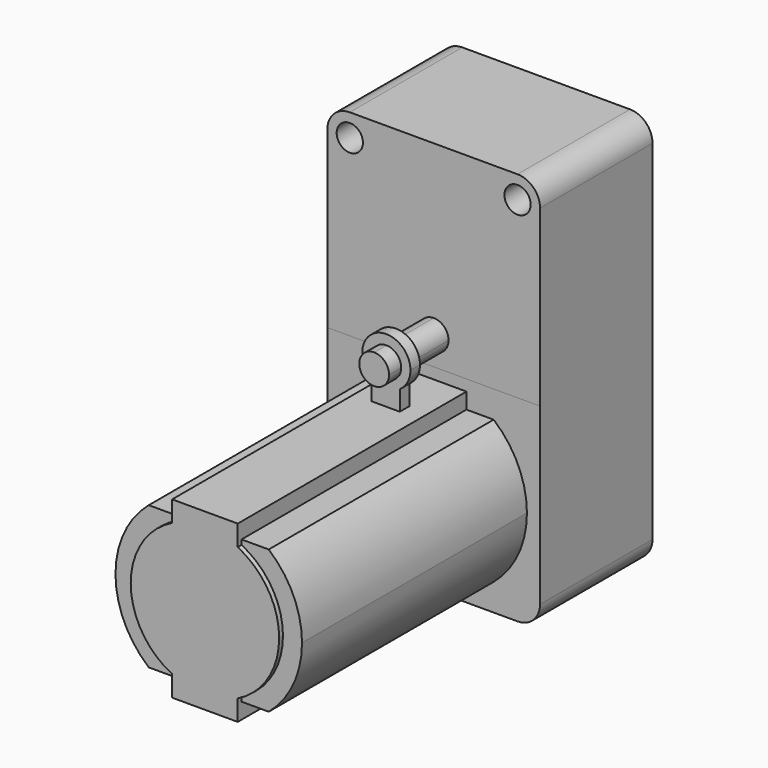
from build123d import *

# Parameters (mm, degrees)
F0_W      = 22.7
F0_H      = 15
F1_DEPTH  = 42
F0_H_2    = 30
F2_DEPTH  = 21
F4_DEPTH  = 7.9375
F5_R      = 2.4
F8_DEPTH  = 29.99994
F11_DEPTH = 1.27
F12_R     = 2.3876
F13_DEPTH = 8.001
F14_DEPTH = 0.762
F6_R      = 1.4
F15_DEPTH = 25.4
F16_DEPTH = 0.508


# Not quite as in the source:
# - a length typed as a fraction of an inch, garbled in the dataset ("3 / 203.2 mm" for 3/8 in), is restored


with BuildPart() as f1:
    # F0 (on Top) → F1 (new body)
    with BuildSketch(Plane.XY):
        with Locations((0, 15)):
            Rectangle(F0_W, F0_H)
    extrude(amount=F1_DEPTH)

    # F0 (on Top) → F2 (join)
    with BuildSketch(Plane.XY):
        with Locations((0, 15)):
            Rectangle(F0_W, F0_H)
        with Locations((0, -7.5)):
            Rectangle(F0_W, F0_H_2)
    extrude(amount=F2_DEPTH)

    # F3 (on face) → F4 (join)
    with BuildSketch(Plane.XZ.offset(-7.5)):
        with BuildLine():
            Line((0, 25.5875), (0, 22.4125))
            ThreePointArc((0, 22.4125), (1.1225320151, 22.8774679849), (1.5875, 24))
            ThreePointArc((1.5875, 24), (1.1225320151, 25.1225320151), (0, 25.5875))
        make_face()
        with BuildLine():
            ThreePointArc((0, 25.5875), (-1.5875, 24), (0, 22.4125))
            Line((0, 22.4125), (0, 25.5875))
        make_face()
    extrude(amount=F4_DEPTH)

    # F5
    f5_edges = [f1.edges().sort_by_distance(p)[0] for p in [
        (-11.35, 15, 42),
        (11.35, 15, 42),
    ]]
    fillet(f5_edges, radius=F5_R)

    # F7 (on face) → F8 (cut)
    with BuildSketch(Plane.XZ.offset(22.5)):
        with BuildLine():
            Line((11.35, 21), (0, 21))
            Line((0, 21), (0, 20.45045))
            ThreePointArc((0, 20.45045), (1.7780416897, 20.2903024954), (3.49885, 19.8150149694))
            ThreePointArc((3.49885, 19.8150149694), (5.0209631758, 19.0907731893), (6.3989886078, 18.12))
            ThreePointArc((6.3989886078, 18.12), (9.0189875095, 14.7034889681), (9.95045, 10.5))
            Line((9.95045, 10.5), (11.35, 10.5))
            Line((11.35, 10.5), (11.35, 21))
        make_face()
        with BuildLine():
            Line((0, 20.45045), (0, 21))
            Line((0, 21), (-11.35, 21))
            Line((-11.35, 21), (-11.35, 10.5))
            Line((-11.35, 10.5), (-9.95045, 10.5))
            ThreePointArc((-9.95045, 10.5), (-9.0189875095, 14.7034889681), (-6.3989886078, 18.12))
            ThreePointArc((-6.3989886078, 18.12), (-5.0209631758, 19.0907731893), (-3.49885, 19.8150149694))
            ThreePointArc((-3.49885, 19.8150149694), (-1.7780416897, 20.2903024954), (0, 20.45045))
        make_face()
        with BuildLine():
            Line((-3.49885, 18.12), (-3.49885, 19.8150149694))
            ThreePointArc((-3.49885, 19.8150149694), (-5.0209631758, 19.0907731893), (-6.3989886078, 18.12))
            Line((-6.3989886078, 18.12), (-3.49885, 18.12))
        make_face()
        with BuildLine():
            ThreePointArc((6.3989886078, 18.12), (5.0209631758, 19.0907731893), (3.49885, 19.8150149694))
            Line((3.49885, 19.8150149694), (3.49885, 18.12))
            Line((3.49885, 18.12), (6.3989886078, 18.12))
        make_face()
        with BuildLine():
            Line((-9.95045, 10.5), (-11.35, 10.5))
            Line((-11.35, 10.5), (-11.35, 0))
            Line((-11.35, 0), (0, 0))
            Line((0, 0), (0, 0.54955))
            ThreePointArc((0, 0.54955), (-1.7780416897, 0.7096975046), (-3.49885, 1.1849850306))
            ThreePointArc((-3.49885, 1.1849850306), (-5.0209631758, 1.9092268107), (-6.3989886078, 2.88))
            ThreePointArc((-6.3989886078, 2.88), (-9.0189875095, 6.2965110319), (-9.95045, 10.5))
        make_face()
        with BuildLine():
            Line((11.35, 0), (11.35, 10.5))
            Line((11.35, 10.5), (9.95045, 10.5))
            ThreePointArc((9.95045, 10.5), (9.0189875095, 6.2965110319), (6.3989886078, 2.88))
            ThreePointArc((6.3989886078, 2.88), (5.0209631758, 1.9092268107), (3.49885, 1.1849850306))
            ThreePointArc((3.49885, 1.1849850306), (1.7780416897, 0.7096975046), (0, 0.54955))
            Line((0, 0.54955), (0, 0))
            Line((0, 0), (11.35, 0))
        make_face()
        with BuildLine():
            ThreePointArc((3.49885, 1.1849850306), (5.0209631758, 1.9092268107), (6.3989886078, 2.88))
            Line((6.3989886078, 2.88), (3.49885, 2.88))
            Line((3.49885, 2.88), (3.49885, 1.1849850306))
        make_face()
        with BuildLine():
            Line((-3.49885, 2.88), (-6.3989886078, 2.88))
            ThreePointArc((-6.3989886078, 2.88), (-5.0209631758, 1.9092268107), (-3.49885, 1.1849850306))
            Line((-3.49885, 1.1849850306), (-3.49885, 2.88))
        make_face()
        with BuildLine():
            ThreePointArc((3.49885, 19.8150149694), (1.7780416897, 20.2903024954), (0, 20.45045))
            Line((0, 20.45045), (0, 19.8150149694))
            Line((0, 19.8150149694), (3.49885, 19.8150149694))
        make_face()
        with BuildLine():
            Line((0, 19.8150149694), (0, 20.45045))
            ThreePointArc((0, 20.45045), (-1.7780416897, 20.2903024954), (-3.49885, 19.8150149694))
            Line((-3.49885, 19.8150149694), (0, 19.8150149694))
        make_face()
        with BuildLine():
            ThreePointArc((0, 0.54955), (1.7780416897, 0.7096975046), (3.49885, 1.1849850306))
            Line((3.49885, 1.1849850306), (0, 1.1849850306))
            Line((0, 1.1849850306), (0, 0.54955))
        make_face()
        with BuildLine():
            ThreePointArc((-3.49885, 1.1849850306), (-1.7780416897, 0.7096975046), (0, 0.54955))
            Line((0, 0.54955), (0, 1.1849850306))
            Line((0, 1.1849850306), (-3.49885, 1.1849850306))
        make_face()
    extrude(amount=-F8_DEPTH, mode=Mode.SUBTRACT)

    # F10 (on offset) → F11 (join)
    with BuildSketch(Plane.XZ.offset(-2.4581)):
        with BuildLine():
            ThreePointArc((1.4326738892, 21.9412771473), (2.2677347419, 22.8658808954), (2.5697519674, 24.0746010095))
            ThreePointArc((2.5697519674, 24.0746010095), (-1.1220643914, 26.3864393852), (-1.5898686834, 22.0557045923))
            Line((-1.5898686834, 22.0557045923), (-1.5898686834, 23.8072182983))
            Line((-1.5898686834, 23.8072182983), (1.4326738892, 23.8072182983))
            Line((1.4326738892, 23.8072182983), (1.4326738892, 21.9412771473))
        make_face()
        with BuildLine():
            Line((-1.5898686834, 23.8072182983), (-1.5898686834, 22.0557045923))
            ThreePointArc((-1.5898686834, 22.0557045923), (-0.0972160525, 21.5066885864), (1.4326738892, 21.9412771473))
            Line((1.4326738892, 21.9412771473), (1.4326738892, 23.8072182983))
            Line((1.4326738892, 23.8072182983), (-1.5898686834, 23.8072182983))
        make_face()
        with BuildLine():
            ThreePointArc((1.4326738892, 21.9412771473), (-0.0972160525, 21.5066885864), (-1.5898686834, 22.0557045923))
            Line((-1.5898686834, 22.0557045923), (-1.5898686834, 19.2958321422))
            Line((-1.5898686834, 19.2958321422), (1.4326738892, 19.2958321422))
            Line((1.4326738892, 19.2958321422), (1.4326738892, 21.9412771473))
        make_face()
    extrude(amount=F11_DEPTH)

    # F12
    f12_edges = [f1.edges().sort_by_distance(p)[0] for p in [
        (11.35, 14.99997, 0),
        (-11.35, 14.99997, 0),
    ]]
    fillet(f12_edges, radius=F12_R)

    # F6 (on face) → F13 (join)
    with BuildSketch(Plane(origin=(0, 22.5, 0), x_dir=(-1, 0, 0), z_dir=(0, 1, 0))):
        with BuildLine():
            ThreePointArc((1.86055, 32.8250564677), (0.9983973943, 33.3623627072), (0, 33.55))
            Line((0, 33.55), (0, 28.05))
            ThreePointArc((0, 28.05), (0.9983973943, 28.2376372928), (1.86055, 28.7749435323))
            Line((1.86055, 28.7749435323), (1.86055, 32.8250564677))
        make_face()
        with BuildLine():
            Line((0, 28.05), (0, 33.55))
            ThreePointArc((0, 33.55), (-0.9983973943, 33.3623627072), (-1.86055, 32.8250564677))
            Line((-1.86055, 32.8250564677), (-1.86055, 28.7749435323))
            ThreePointArc((-1.86055, 28.7749435323), (-0.9983973943, 28.2376372928), (0, 28.05))
        make_face()
    extrude(amount=F13_DEPTH)

    # F6 (on face) → F14 (join)
    with BuildSketch(Plane(origin=(0, 22.5, 0), x_dir=(-1, 0, 0), z_dir=(0, 1, 0))):
        with BuildLine():
            ThreePointArc((3.3400836906, 30.8), (2.3617958273, 33.1617958273), (0, 34.1400836906))
            Line((0, 34.1400836906), (0, 33.55))
            ThreePointArc((0, 33.55), (0.9983973943, 33.3623627072), (1.86055, 32.8250564677))
            ThreePointArc((1.86055, 32.8250564677), (2.5178376139, 31.9058904783), (2.75, 30.8))
            ThreePointArc((2.75, 30.8), (2.5178376139, 29.6941095217), (1.86055, 28.7749435323))
            ThreePointArc((1.86055, 28.7749435323), (0.9983973943, 28.2376372928), (0, 28.05))
            Line((0, 28.05), (0, 27.4599163094))
            ThreePointArc((0, 27.4599163094), (2.3617958273, 28.4382041727), (3.3400836906, 30.8))
        make_face()
        with BuildLine():
            Line((0, 33.55), (0, 34.1400836906))
            ThreePointArc((0, 34.1400836906), (-3.3400836906, 30.8), (0, 27.4599163094))
            Line((0, 27.4599163094), (0, 28.05))
            ThreePointArc((0, 28.05), (-0.9983973943, 28.2376372928), (-1.86055, 28.7749435323))
            ThreePointArc((-1.86055, 28.7749435323), (-2.75, 30.8), (-1.86055, 32.8250564677))
            ThreePointArc((-1.86055, 32.8250564677), (-0.9983973943, 33.3623627072), (0, 33.55))
        make_face()
    extrude(amount=F14_DEPTH)

    # F6 (on face) → F15 (cut)
    with BuildSketch(Plane(origin=(0, 22.5, 0), x_dir=(-1, 0, 0), z_dir=(0, 1, 0))):
        with Locations((-8.95, 39.6)):
            Circle(F6_R)
        with Locations((8.95, 39.6)):
            Circle(F6_R)
    extrude(amount=-F15_DEPTH, mode=Mode.SUBTRACT)

    # F7 (on face) → F16 (join)
    with BuildSketch(Plane.XZ.offset(22.5)):
        with BuildLine():
            ThreePointArc((7.91845, 10.5), (6.7233666859, 14.6830838875), (3.49885, 17.6035131505))
            Line((3.49885, 17.6035131505), (3.49885, 10.5))
            Line((3.49885, 10.5), (7.91845, 10.5))
        make_face()
        with BuildLine():
            Line((2.1534740311, 18.12), (0, 18.12))
            Line((0, 18.12), (0, 10.5))
            Line((0, 10.5), (3.49885, 10.5))
            Line((3.49885, 10.5), (3.49885, 17.6035131505))
            ThreePointArc((3.49885, 17.6035131505), (2.8379361171, 17.8924264621), (2.1534740311, 18.12))
        make_face()
        with BuildLine():
            Line((0, 10.5), (0, 18.12))
            Line((0, 18.12), (-2.1534740311, 18.12))
            ThreePointArc((-2.1534740311, 18.12), (-2.8379361171, 17.8924264621), (-3.49885, 17.6035131505))
            Line((-3.49885, 17.6035131505), (-3.49885, 10.5))
            Line((-3.49885, 10.5), (0, 10.5))
        make_face()
        with BuildLine():
            Line((-3.49885, 10.5), (-3.49885, 17.6035131505))
            ThreePointArc((-3.49885, 17.6035131505), (-6.7233666859, 14.6830838875), (-7.91845, 10.5))
            Line((-7.91845, 10.5), (-3.49885, 10.5))
        make_face()
        with BuildLine():
            Line((-3.49885, 10.5), (-7.91845, 10.5))
            ThreePointArc((-7.91845, 10.5), (-6.7233666859, 6.3169161125), (-3.49885, 3.3964868495))
            Line((-3.49885, 3.3964868495), (-3.49885, 10.5))
        make_face()
        with BuildLine():
            Line((0, 2.88), (0, 10.5))
            Line((0, 10.5), (-3.49885, 10.5))
            Line((-3.49885, 10.5), (-3.49885, 3.3964868495))
            ThreePointArc((-3.49885, 3.3964868495), (-2.8379361171, 3.1075735379), (-2.1534740311, 2.88))
            Line((-2.1534740311, 2.88), (0, 2.88))
        make_face()
        with BuildLine():
            Line((3.49885, 10.5), (0, 10.5))
            Line((0, 10.5), (0, 2.88))
            Line((0, 2.88), (2.1534740311, 2.88))
            ThreePointArc((2.1534740311, 2.88), (2.8379361171, 3.1075735379), (3.49885, 3.3964868495))
            Line((3.49885, 3.3964868495), (3.49885, 10.5))
        make_face()
        with BuildLine():
            ThreePointArc((3.49885, 3.3964868495), (6.7233666859, 6.3169161125), (7.91845, 10.5))
            Line((7.91845, 10.5), (3.49885, 10.5))
            Line((3.49885, 10.5), (3.49885, 3.3964868495))
        make_face()
        with BuildLine():
            ThreePointArc((2.1534740311, 18.12), (1.0870283811, 18.3434826258), (0, 18.41845))
            Line((0, 18.41845), (0, 18.12))
            Line((0, 18.12), (2.1534740311, 18.12))
        make_face()
        with BuildLine():
            Line((0, 18.12), (0, 18.41845))
            ThreePointArc((0, 18.41845), (-1.0870283811, 18.3434826258), (-2.1534740311, 18.12))
            Line((-2.1534740311, 18.12), (0, 18.12))
        make_face()
        with BuildLine():
            Line((2.1534740311, 2.88), (0, 2.88))
            Line((0, 2.88), (0, 2.58155))
            ThreePointArc((0, 2.58155), (1.0870283811, 2.6565173742), (2.1534740311, 2.88))
        make_face()
        with BuildLine():
            Line((0, 2.58155), (0, 2.88))
            Line((0, 2.88), (-2.1534740311, 2.88))
            ThreePointArc((-2.1534740311, 2.88), (-1.0870283811, 2.6565173742), (0, 2.58155))
        make_face()
        with BuildLine():
            Line((3.49885, 19.8150149694), (0, 19.8150149694))
            Line((0, 19.8150149694), (0, 18.41845))
            ThreePointArc((0, 18.41845), (1.0870283811, 18.3434826258), (2.1534740311, 18.12))
            Line((2.1534740311, 18.12), (3.49885, 18.12))
            Line((3.49885, 18.12), (3.49885, 19.8150149694))
        make_face()
        with BuildLine():
            Line((0, 18.41845), (0, 19.8150149694))
            Line((0, 19.8150149694), (-3.49885, 19.8150149694))
            Line((-3.49885, 19.8150149694), (-3.49885, 18.12))
            Line((-3.49885, 18.12), (-2.1534740311, 18.12))
            ThreePointArc((-2.1534740311, 18.12), (-1.0870283811, 18.3434826258), (0, 18.41845))
        make_face()
        with BuildLine():
            Line((-2.1534740311, 18.12), (-3.49885, 18.12))
            Line((-3.49885, 18.12), (-3.49885, 17.6035131505))
            ThreePointArc((-3.49885, 17.6035131505), (-2.8379361171, 17.8924264621), (-2.1534740311, 18.12))
        make_face()
        with BuildLine():
            Line((3.49885, 17.6035131505), (3.49885, 18.12))
            Line((3.49885, 18.12), (2.1534740311, 18.12))
            ThreePointArc((2.1534740311, 18.12), (2.8379361171, 17.8924264621), (3.49885, 17.6035131505))
        make_face()
        with BuildLine():
            Line((0, 1.1849850306), (3.49885, 1.1849850306))
            Line((3.49885, 1.1849850306), (3.49885, 2.88))
            Line((3.49885, 2.88), (2.1534740311, 2.88))
            ThreePointArc((2.1534740311, 2.88), (1.0870283811, 2.6565173742), (0, 2.58155))
            Line((0, 2.58155), (0, 1.1849850306))
        make_face()
        with BuildLine():
            Line((-3.49885, 2.88), (-3.49885, 1.1849850306))
            Line((-3.49885, 1.1849850306), (0, 1.1849850306))
            Line((0, 1.1849850306), (0, 2.58155))
            ThreePointArc((0, 2.58155), (-1.0870283811, 2.6565173742), (-2.1534740311, 2.88))
            Line((-2.1534740311, 2.88), (-3.49885, 2.88))
        make_face()
        with BuildLine():
            ThreePointArc((-2.1534740311, 2.88), (-2.8379361171, 3.1075735379), (-3.49885, 3.3964868495))
            Line((-3.49885, 3.3964868495), (-3.49885, 2.88))
            Line((-3.49885, 2.88), (-2.1534740311, 2.88))
        make_face()
        with BuildLine():
            Line((3.49885, 2.88), (3.49885, 3.3964868495))
            ThreePointArc((3.49885, 3.3964868495), (2.8379361171, 3.1075735379), (2.1534740311, 2.88))
            Line((2.1534740311, 2.88), (3.49885, 2.88))
        make_face()
    extrude(amount=F16_DEPTH)


solid = f1.part
